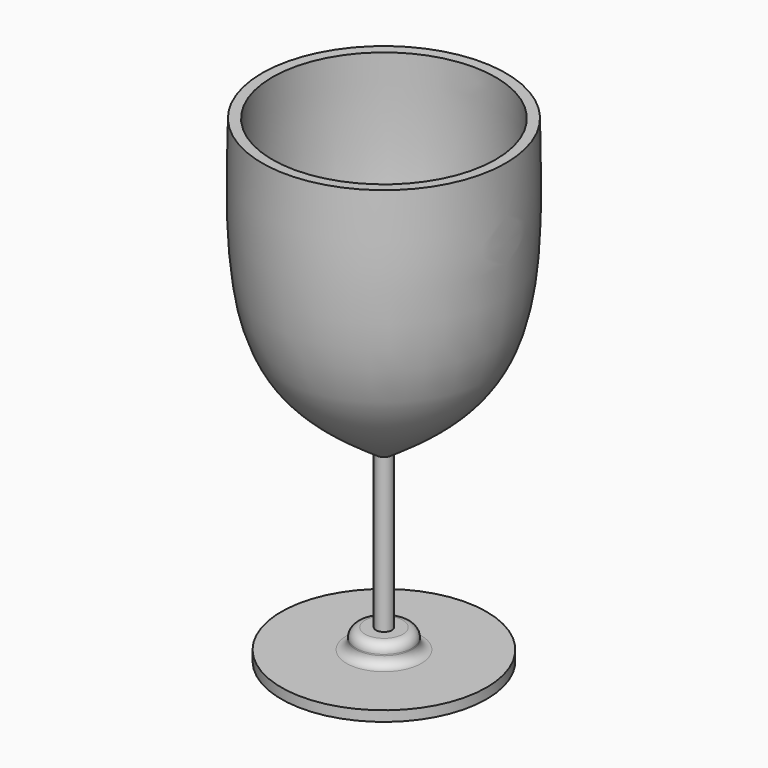
from build123d import *

# Parameters (mm, degrees)
F2_R = 2.286


# Not quite as in the source:
# - the dataset's text gives a spline's control points without its knots; the knots are read off the source's solid


with BuildPart() as f1:
    # F0 (on Front) → F1 (revolve)
    with BuildSketch(Plane.XZ):
        with BuildLine():
            Line((0, 47.6139092823), (0, 0))
            Line((0, 0), (25.4, 0))
            Line((25.4, 0), (25.4, 2.54))
            Line((25.4, 2.54), (6.9723119959, 2.54))
            Line((6.9723119959, 2.54), (6.9723119959, 7.4226073921))
            Line((6.9723119959, 7.4226073921), (1.9854572602, 7.4226073921))
            Line((1.9854572602, 7.4226073921), (1.9854572602, 45.5226073921))
            add(Edge.make_bspline(
                [(1.9854572602, 45.5226073921), (9.1183458915, 50.4393489291), (22.9946563844, 60.0043702981), (30.9719457485, 82.3906969255), (30.4589425939, 105.4166327755), (30.1707796752, 118.3507069945)],
                knots=[0, 0, 0, 0, 0.3167510601, 0.6162070217, 1, 1, 1, 1], degree=3))
            Line((30.1707796752, 118.3507069945), (27.6314098305, 118.2941314551))
            add(Edge.make_bspline(
                [(0.5439107281, 47.6139092823), (1.9513426061, 48.5840602454), (4.7520594595, 50.514716622), (8.8009190581, 53.4309124613), (12.587142562, 56.4115346213), (15.431990129, 58.9806996874), (17.4700514796, 61.1037584309), (18.8670813382, 62.7321741187), (20.1249479639, 64.4060497761), (21.6403604896, 66.724897673), (23.2471186454, 69.7952235715), (24.7728044852, 73.8098530535), (25.9405021256, 78.1988066628), (26.7913628714, 82.9987097248), (27.3671494468, 88.2289946642), (27.8215961355, 95.6718703705), (27.9122878106, 105.6813195614), (27.7252634622, 114.0815497541), (27.6314098305, 118.2941314551)],
                knots=[-3e-10, -3e-10, -3e-10, -3e-10, 0.0624999997, 0.1249999998, 0.1874999998, 0.2499999998, 0.2812499998, 0.3124999998, 0.3437499998, 0.3749999998, 0.4374999998, 0.4999999999, 0.5624999999, 0.6249999999, 0.6874999999, 0.7499999999, 0.875, 1, 1, 1, 1], degree=3))
            Line((0.5439107281, 47.6139092823), (0, 47.6139092823))
        make_face()
    revolve(axis=Axis((0, 0, 23.8069546411), (0, 0, -1)))

    # F2
    f2_edges = [f1.edges().sort_by_distance(p)[0] for p in [
        (-6.972312, 0, 7.422607),
        (-6.972312, 0, 2.54),
    ]]
    fillet(f2_edges, radius=F2_R)


solid = f1.part
